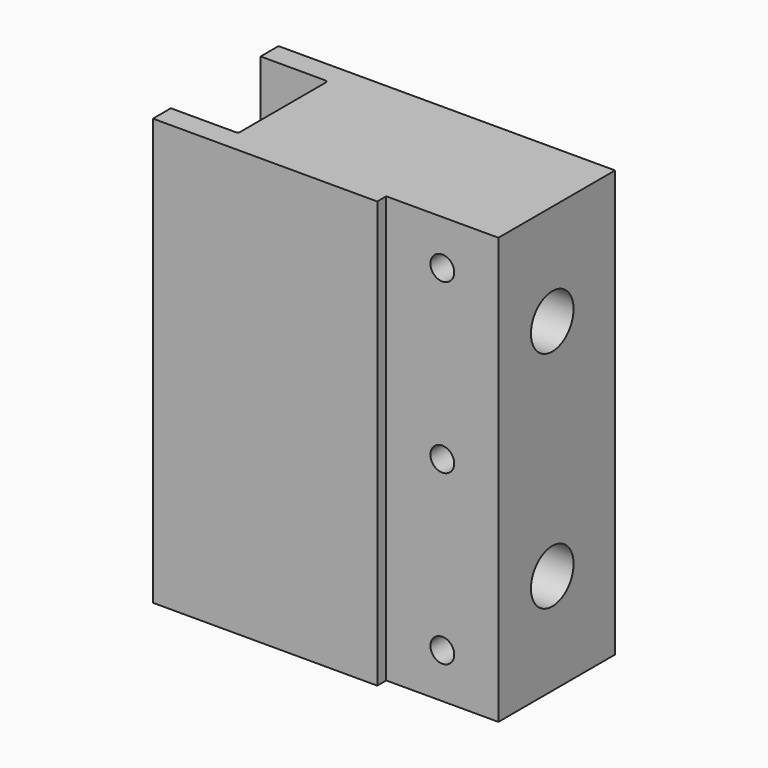
from build123d import *

# Parameters (mm, degrees)
F1_DEPTH       = 120.65
F2_R           = 1.524
F4_D           = 20.6375
F4_CBORE_D     = 30.1752
F4_CBORE_DEPTH = 28.448
F5_W           = 63.5
F5_H           = 241.3
F6_DEPTH       = 6.35
F8_D           = 13.49248
F8_DEPTH       = 41.2172727273
F8_TIP         = 4.0535499425


# Not quite as in the source:
# - a length typed as a fraction of an inch, garbled in the dataset ("3 / 203.2 mm" for 3/8 in), is restored


with BuildPart() as f1:
    # F0 (on Top) → F1 (new body, symmetric)
    with BuildSketch(Plane.XY):
        Polygon((95.25, 44.45), (-95.25, 44.45), (-95.25, 31.75), (-57.15, 31.75), (-57.15, -31.75), (-95.25, -31.75), (-95.25, -44.45), (95.25, -44.45), align=None)
    extrude(amount=F1_DEPTH, both=True)

    # F2
    f2_edges = [f1.edges().sort_by_distance(p)[0] for p in [
        (-57.15, 31.75, 0),
        (-57.15, -31.75, 0),
    ]]
    fillet(f2_edges, radius=F2_R)

    # F4 (through all)
    with Locations(Plane.YZ.offset(95.25)):
        with Locations((0, 63.5), (0, -63.5)):
            CounterBoreHole(F4_D / 2, F4_CBORE_D / 2, F4_CBORE_DEPTH)

    # F5 (on face) → F6 (cut)
    with BuildSketch(Plane.XZ.offset(44.45)):
        with Locations((63.5, 0)):
            Rectangle(F5_W, F5_H)
    extrude(amount=-F6_DEPTH, mode=Mode.SUBTRACT)

    # F8
    with Locations(Plane.XZ.offset(38.1)):
        with Locations((63.5, 95.25), (63.5, 0), (63.5, -95.25)):
            Hole(F8_D / 2, depth=F8_DEPTH)
            with Locations((0, 0, -(F8_DEPTH + F8_TIP / 2))):  # 118° drill point
                Cone(0, F8_D / 2, F8_TIP, mode=Mode.SUBTRACT)


solid = f1.part
